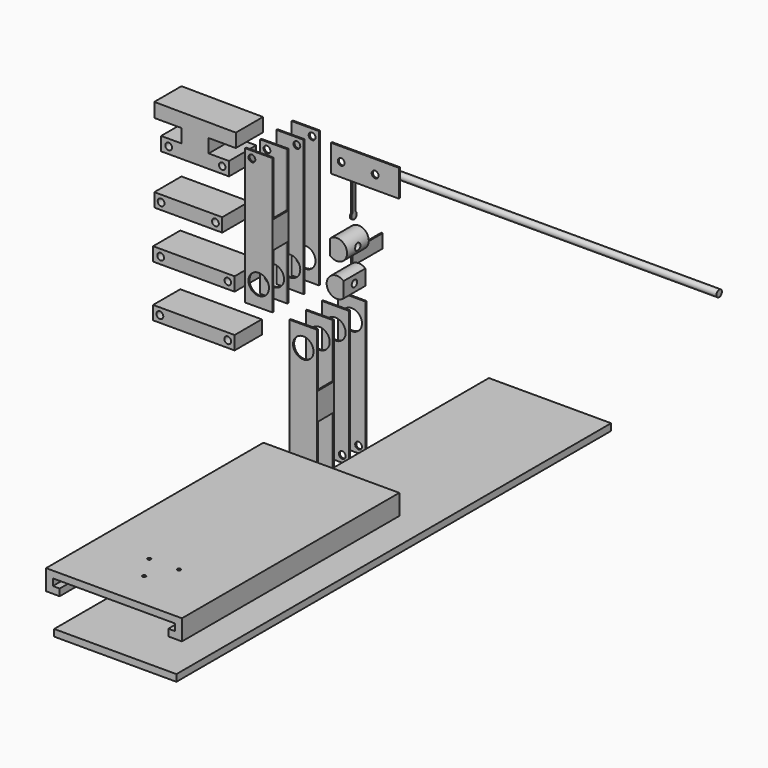
from build123d import *

# Parameters (mm, degrees)
F1_DEPTH  = 100
F2_R      = 7.5
F2_R_2    = 2.5
F3_DEPTH  = 15.001
F4_W      = 13
F4_H      = 40
F5_DEPTH  = 20.1627097718
F6_DEPTH  = 100
F7_R      = 7.5
F7_R_2    = 2.5
F8_DEPTH  = 16.001
F9_W      = 14
F9_H      = 40
F10_DEPTH = 20.1691592966
F11_W     = 50
F11_H     = 20
F11_R     = 2.5
F12_DEPTH = 1
F13_R     = 2.5
F13_R_2   = 7.5
F14_DEPTH = 45.1330833913
F15_R     = 7.5
F15_R_2   = 2.5
F16_DEPTH = 46.1330833913
F17_W     = 14
F17_H     = 40
F18_DEPTH = 53.5847666336
F19_W     = 13
F19_H     = 40
F20_DEPTH = 25
F22_DEPTH = 20
F23_R     = 2.5
F24_DEPTH = 250
F25_W     = 50
F25_H     = 10
F25_R     = 2.5
F26_DEPTH = 25
F25_R_2   = 2.4144593705
F25_W_2   = 60
F27_DEPTH = 25
F28_R     = 2.5
F29_DEPTH = 136.2251037518
F30_R     = 2.5
F31_DEPTH = 214.5146418358
F33_DEPTH = 1
F34_W     = 1
F34_H     = 10
F35_DEPTH = 25
F37_DEPTH = 400
F38_R     = 1.25
F39_DEPTH = 83.0761684308
F40_W     = 100
F40_H     = 200
F41_DEPTH = 127.4896658788


# Not quite as in the source:
# - a feature names something its author has since deleted; it is built from what else it names


with BuildPart() as f1:
    # F0 (on Top) → F1 (new body)
    with BuildSketch(Plane.XY):
        Polygon((0, 14), (0, 15), (-20, 15), (-20, 0), (0, 0), (0, 1), (-19, 1), (-19, 14), align=None)
    extrude(amount=F1_DEPTH)

    # F2 (on face) → F3 (cut, through all)
    with BuildSketch(Plane.XZ):
        with Locations((-10, 15)):
            Circle(F2_R)
        with Locations((-5, 95)):
            Circle(F2_R_2)
    extrude(amount=-F3_DEPTH, mode=Mode.SUBTRACT)

    # F4 (on face) → F5 (cut, through all)
    with BuildSketch(Plane(origin=(-20, 0, 0), x_dir=(0, -1, 0), z_dir=(-1, 0, 0))):
        with Locations((-7.5, 20)):
            Rectangle(F4_W, F4_H)
        with Locations((-7.5, 80)):
            Rectangle(F4_W, F4_H)
    extrude(amount=-F5_DEPTH, mode=Mode.SUBTRACT)


with BuildPart() as f1b:
    # F0 (on Top) → F1, piece 2 (new body)
    with BuildSketch(Plane.XY):
        Polygon((0.051417134, -13.985459061), (-19.9480422158, -14.1325159114), (-19.9406893732, -15.1324888789), (-0.941202991, -14.992784871), (-0.8456160382, -27.9924334484), (-19.837749578, -28.1320833905), (-19.837749578, -29.1321104238), (0.1617097718, -28.9850535734), align=None)
    extrude(amount=F1_DEPTH)

    # F13 (on face) → F14 (cut, through all)
    with BuildSketch(Plane(origin=(0.2131255159, -28.9846755113, 0), x_dir=(0.9999729675, 0.0073528425, 0), z_dir=(0.0073528425, -0.9999729675, 0))):
        with Locations((-15.051417134, 95)):
            Circle(F13_R)
        with Locations((-10.051417134, 15)):
            Circle(F13_R_2)
    extrude(amount=-F14_DEPTH, mode=Mode.SUBTRACT)

    # F19 (on face) → F20 (cut)
    with BuildSketch(Plane(origin=(-0.0514157441, -0.0003780621, 0), x_dir=(-0.0073528425, 0.9999729675, 0), z_dir=(0.9999729675, 0.0073528425, 0))):
        with Locations((-21.485459061, 20)):
            Rectangle(F19_W, F19_H)
        with Locations((-21.485459061, 80)):
            Rectangle(F19_W, F19_H)
    extrude(amount=-F20_DEPTH, mode=Mode.SUBTRACT)


with BuildPart() as f6:
    # F0 (on Top) → F6 (new body)
    with BuildSketch(Plane.XY):
        Polygon((33.4159745649, 0), (33.4159745649, 1), (14.4159745649, 1), (14.4159745649, 15), (33.4159745649, 15), (33.4159745649, 16), (13.4159745649, 16), (13.4159745649, 0), align=None)
    extrude(amount=-F6_DEPTH)

    # F7 (on face) → F8 (cut, through all)
    with BuildSketch(Plane.XZ):
        with Locations((23.4159745649, -15)):
            Circle(F7_R)
        with Locations((28.4159745649, -95)):
            Circle(F7_R_2)
    extrude(amount=-F8_DEPTH, mode=Mode.SUBTRACT)

    # F9 (on face) → F10 (cut, through all)
    with BuildSketch(Plane(origin=(13.4159745649, 0, 0), x_dir=(0, -1, 0), z_dir=(-1, 0, 0))):
        with Locations((-8, -20)):
            Rectangle(F9_W, F9_H)
        with Locations((-8, -80)):
            Rectangle(F9_W, F9_H)
    extrude(amount=-F10_DEPTH, mode=Mode.SUBTRACT)


with BuildPart() as f6b:
    # F0 (on Top) → F6, piece 2 (new body)
    with BuildSketch(Plane.XY):
        Polygon((33.4664883811, -13.7397566624), (13.4670290313, -13.8868135128), (13.4743818739, -14.8867864803), (32.4738682561, -14.7470824724), (32.5768080514, -28.7467040172), (13.5846745117, -28.8863539594), (13.5846745117, -29.8863809926), (33.5841338614, -29.7393241422), align=None)
    extrude(amount=-F6_DEPTH)

    # F15 (on face) → F16 (cut, through all)
    with BuildSketch(Plane(origin=(0.2204783584, -29.9846484788, 0), x_dir=(0.9999729675, 0.0073528425, 0), z_dir=(0.0073528425, -0.9999729675, 0))):
        with Locations((23.3645574309, -15)):
            Circle(F15_R)
        with Locations((18.3645574309, -95)):
            Circle(F15_R_2)
    extrude(amount=-F16_DEPTH, mode=Mode.SUBTRACT)

    # F17 (on face) → F18 (cut, through all)
    with BuildSketch(Plane(origin=(33.3636555031, 0.2453243365, 0), x_dir=(-0.0073528425, 0.9999729675, 0), z_dir=(0.9999729675, 0.0073528425, 0))):
        with Locations((-21.985459061, -20)):
            Rectangle(F17_W, F17_H)
        with Locations((-21.985459061, -80)):
            Rectangle(F17_W, F17_H)
    extrude(amount=-F18_DEPTH, mode=Mode.SUBTRACT)


with BuildPart() as f12:
    # F11 (on Front) → F12 (new body)
    with BuildSketch(Plane.XZ):
        with Locations((45.8931141218, 95.3558683395)):
            Rectangle(F11_W, F11_H)
        with Locations((28.3931141218, 95.3558683395)):
            Circle(F11_R, mode=Mode.SUBTRACT)
        with Locations((53.3931141218, 95.3558683395)):
            Circle(F11_R, mode=Mode.SUBTRACT)
    extrude(amount=F12_DEPTH)


with BuildPart() as f22:
    # F21 (on Front) → F22 (new body)
    with BuildSketch(Plane.XZ):
        with BuildLine():
            Line((35.4863581642, 55.8813297105), (35.4863581642, 44.6073331245))
            ThreePointArc((35.4863581642, 44.6073331245), (47.9335038306, 50.2443314175), (35.4863581642, 55.8813297105))
        make_face()
    extrude(amount=F22_DEPTH)

    # F30 (on face) → F31 (cut, through all)
    with BuildSketch(Plane(origin=(35.4863581642, 0, 0), x_dir=(0, -1, 0), z_dir=(-1, 0, 0))):
        with Locations((10, 50.2443314175)):
            Circle(F30_R)
    extrude(amount=-F31_DEPTH, mode=Mode.SUBTRACT)


with BuildPart() as f22b:
    # F21 (on Front) → F22, piece 2 (new body)
    with BuildSketch(Plane.XZ):
        with BuildLine():
            Line((45.380649497, 20.1312099156), (45.380649497, 31.4052065016))
            ThreePointArc((45.380649497, 31.4052065016), (32.9335038306, 25.7682082086), (45.380649497, 20.1312099156))
        make_face()
    extrude(amount=F22_DEPTH)

    # F28 (on face) → F29 (cut, through all)
    with BuildSketch(Plane.YZ.offset(45.380649497)):
        with Locations((-10, 25.7682082086)):
            Circle(F28_R)
    extrude(amount=-F29_DEPTH, mode=Mode.SUBTRACT)


with BuildPart() as f24:
    # F23 (on Right) → F24 (new body)
    with BuildSketch(Plane.YZ):
        with Locations((69.883659482, 53.4276850522)):
            Circle(F23_R)
    extrude(amount=F24_DEPTH)


with BuildPart() as f26:
    # F25 (on Front) → F26 (new body)
    with BuildSketch(Plane.XZ):
        with Locations((-64.9493469292, 42.0624911785)):
            Rectangle(F25_W, F25_H)
        with Locations((-84.9493469292, 42.0624911785)):
            Circle(F25_R, mode=Mode.SUBTRACT)
        with Locations((-44.9493469292, 42.0624911785)):
            Circle(F25_R, mode=Mode.SUBTRACT)
    extrude(amount=F26_DEPTH)


with BuildPart() as f26b:
    # F25 (on Front) → F26, piece 2 (new body)
    with BuildSketch(Plane.XZ):
        Polygon((-84.9493469292, 85.124527216), (-84.9493469292, 75.124527216), (-34.9493469292, 75.124527216), (-34.9493469292, 85.124527216), (-49.9493469292, 85.124527216), (-49.9493469292, 95.124527216), (-29.9493469292, 95.124527216), (-29.9493469292, 105.124527216), (-89.9493469292, 105.5638343096), (-89.9493469292, 95.124527216), (-69.9493469292, 95.124527216), (-69.9493469292, 85.124527216), align=None)
        with Locations((-79.3778774142, 80.124527216)):
            Circle(F25_R, mode=Mode.SUBTRACT)
        with Locations((-39.9493469292, 80.124527216)):
            Circle(F25_R_2, mode=Mode.SUBTRACT)
    extrude(amount=F26_DEPTH)


with BuildPart() as f27:
    # F25 (on Front) → F27 (new body)
    with BuildSketch(Plane.XZ):
        with Locations((-60.8434542548, -31.3186603598)):
            Rectangle(F25_W_2, F25_H)
        with Locations((-85.8434542548, -31.3186603598)):
            Circle(F25_R, mode=Mode.SUBTRACT)
        with Locations((-35.8434542548, -31.3186603598)):
            Circle(F25_R, mode=Mode.SUBTRACT)
    extrude(amount=F27_DEPTH)


with BuildPart() as f27b:
    # F25 (on Front) → F27, piece 2 (new body)
    with BuildSketch(Plane.XZ):
        with Locations((-60.8434542548, 6.7433756776)):
            Rectangle(F25_W_2, F25_H)
        with Locations((-85.2719847398, 6.7433756776)):
            Circle(F25_R, mode=Mode.SUBTRACT)
        with Locations((-35.8434542548, 6.7433756776)):
            Circle(F25_R_2, mode=Mode.SUBTRACT)
    extrude(amount=F27_DEPTH)


with BuildPart() as f33:
    # F32 (on Right) → F33 (new body)
    with BuildSketch(Plane.YZ):
        with BuildLine():
            Line((47.762863338, 8.6800148711), (47.762863338, 20.4667558931))
            ThreePointArc((47.762863338, 20.4667558931), (46.3052242994, 24.9978365004), (44.8475852609, 20.4667558931))
            Line((44.8475852609, 20.4667558931), (44.8475852609, 8.6800148711))
            Line((44.8475852609, 8.6800148711), (44.8475852609, 0))
            Line((44.8475852609, 0), (47.762863338, 0))
            Line((47.762863338, 0), (47.762863338, 8.6800148711))
        make_face()
    extrude(amount=-F33_DEPTH)

    # F34 (on face) → F35 (join)
    with BuildSketch(Plane(origin=(0, 47.762863338, 0), x_dir=(-1, 0, 0), z_dir=(0, 1, 0))):
        with Locations((0.5, 5)):
            Rectangle(F34_W, F34_H)
    extrude(amount=F35_DEPTH)


with BuildPart() as f33b:
    # F32 (on Right) → F33, piece 2 (new body)
    with BuildSketch(Plane.YZ):
        with BuildLine():
            ThreePointArc((44.8475852609, 34.1576339639), (46.3052242994, 29.6265533566), (47.762863338, 34.1576339639))
            Line((47.762863338, 34.1576339639), (47.762863338, 45.944374986))
            Line((47.762863338, 45.944374986), (47.762863338, 54.6243898571))
            Line((47.762863338, 54.6243898571), (44.8475852609, 54.6243898571))
            Line((44.8475852609, 54.6243898571), (44.8475852609, 45.944374986))
            Line((44.8475852609, 45.944374986), (44.8475852609, 34.1576339639))
        make_face()
    extrude(amount=-F33_DEPTH)


with BuildPart() as f37:
    # F36 (on Front) → F37 (new body)
    with BuildSketch(Plane.XZ):
        Polygon((220.3795283456, 17.4886658788), (220.3795283456, 12.4886658788), (230.3795283456, 12.4886658788), (230.3795283456, 27.4886658788), (180.3795283456, 27.4886658788), (130.3795283456, 27.4886658788), (130.3795283456, 12.4886658788), (140.3795283456, 12.4886658788), (140.3795283456, 17.4886658788), (135.3795283456, 17.4886658788), (135.3795283456, 22.4886658788), (180.3795283456, 22.4886658788), (225.3795283456, 22.4886658788), (225.3795283456, 17.4886658788), align=None)
    extrude(amount=F37_DEPTH)

    # F38 (on face) → F39 (cut, through all)
    with BuildSketch(Plane(origin=(0, 0, 22.4886658788), x_dir=(1, 0, 0), z_dir=(0, 0, -1))):
        with Locations((180.5873862401, 372.4982716843)):
            Circle(F38_R)
        with Locations((169.4517786162, 353.9308743749)):
            Circle(F38_R)
        with Locations((191.0994201803, 353.5708539408)):
            Circle(F38_R)
    extrude(amount=-F39_DEPTH, mode=Mode.SUBTRACT)

    # F40 (on face) → F41 (cut, through all)
    with BuildSketch(Plane.XY.offset(27.4886658788)):
        with Locations((180.3795283456, -100)):
            Rectangle(F40_W, F40_H)
    extrude(amount=-F41_DEPTH, mode=Mode.SUBTRACT)


with BuildPart() as f37b:
    # F36 (on Front) → F37, piece 2 (new body)
    with BuildSketch(Plane.XZ):
        Polygon((136.3347970862, -15.0014664978), (181.3347970862, -15.0014664978), (226.3347970862, -15.0014664978), (226.3347970862, -10.0014664978), (181.3347970862, -10.0014664978), (136.3347970862, -10.0014664978), align=None)
    extrude(amount=F37_DEPTH)


solid = Compound([f1.part, f1b.part, f6.part, f6b.part, f12.part, f22.part, f22b.part, f24.part, f26.part, f26b.part, f27.part, f27b.part, f33.part, f33b.part, f37.part, f37b.part])
